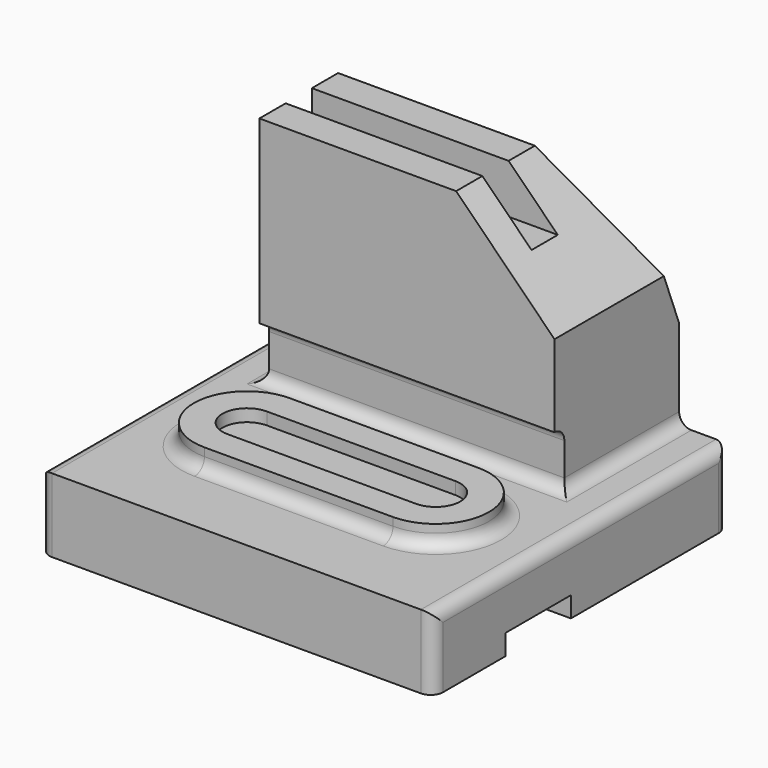
from build123d import *

# Parameters (mm, degrees)
F0_W      = 96
F0_H      = 90
F1_DEPTH  = 18
F2_W      = 72
F2_H      = 38
F4_DEPTH  = 58
F6_DEPTH  = 38
F7_W      = 8
F7_H      = 12
F8_DEPTH  = 60.001
F10_DEPTH = 72.001
F11_W     = 20
F11_H     = 5
F12_DEPTH = 96
F13_W     = 46
F13_H     = 26
F14_DEPTH = 5
F15_W     = 46
F15_H     = 12
F17_DEPTH = 3
F18_W     = 3
F18_H     = 14
F19_DEPTH = 72
F20_R     = 2.99999


# Not quite as in the source:
# - a fillet or chamfer is up to 0.001 mm smaller than in the source, because OpenCascade refuses the exact size


with BuildPart() as f1:
    # F0 (on Top) → F1 (new body)
    with BuildSketch(Plane.XY):
        with Locations((48, 45)):
            Rectangle(F0_W, F0_H)
    extrude(amount=F1_DEPTH)

    # F2 (on face) → F4 (join, through all)
    with BuildSketch(Plane.XY.offset(18)):
        with Locations((48, 71)):
            Rectangle(F2_W, F2_H)
    extrude(amount=F4_DEPTH)

    # F5 (on face) → F6 (cut, through all)
    with BuildSketch(Plane.XZ.offset(-52)):
        Polygon((84, 52), (84, 76), (60, 76), align=None)
    extrude(amount=-F6_DEPTH, mode=Mode.SUBTRACT)

    # F7 (on face) → F8 (cut, through all)
    with BuildSketch(Plane(origin=(12, 0, 0), x_dir=(0, -1, 0), z_dir=(-1, 0, 0))):
        with Locations((-64, 70)):
            Rectangle(F7_W, F7_H)
    extrude(amount=-F8_DEPTH, mode=Mode.SUBTRACT)

    # F9 (on face) → F10 (cut, through all)
    with BuildSketch(Plane(origin=(12, 0, 0), x_dir=(0, -1, 0), z_dir=(-1, 0, 0))):
        Polygon((-90, 40), (-76, 76), (-90, 76), align=None)
    extrude(amount=-F10_DEPTH, mode=Mode.SUBTRACT)

    # F11 (on face) → F12 (cut, through all)
    with BuildSketch(Plane.YZ.offset(96)):
        with Locations((32, 2.5)):
            Rectangle(F11_W, F11_H)
    extrude(amount=-F12_DEPTH, mode=Mode.SUBTRACT)

    # F13 (on face) → F14 (join)
    with BuildSketch(Plane.XY.offset(18)):
        with Locations((48, 31.9999999999)):
            Rectangle(F13_W, F13_H)
        with BuildLine():
            Line((25, 18.9999999999), (25, 44.9999999999))
            ThreePointArc((25, 44.9999999999), (12, 31.9999999999), (25, 18.9999999999))
        make_face()
        with BuildLine():
            ThreePointArc((71, 18.9999999999), (84, 31.9999999999), (71, 44.9999999999))
            Line((71, 44.9999999999), (71, 18.9999999999))
        make_face()
    extrude(amount=F14_DEPTH)

    # F15 (on face) → F17 (cut, through all)
    with BuildSketch(Plane.XY.offset(23)):
        with Locations((48, 31.9999999999)):
            Rectangle(F15_W, F15_H)
        with BuildLine():
            Line((25, 25.9999999999), (25, 37.9999999999))
            ThreePointArc((25, 37.9999999999), (19, 31.9999999999), (25, 25.9999999999))
        make_face()
        with BuildLine():
            ThreePointArc((71, 25.9999999999), (77, 31.9999999999), (71, 37.9999999999))
            Line((71, 37.9999999999), (71, 25.9999999999))
        make_face()
    extrude(amount=-F17_DEPTH, mode=Mode.SUBTRACT)

    # F18 (on face) → F19 (cut, through all)
    with BuildSketch(Plane.YZ.offset(84)):
        with Locations((53.5, 25)):
            Rectangle(F18_W, F18_H)
    extrude(amount=-F19_DEPTH, mode=Mode.SUBTRACT)

    # F20 (radius 3 in the source; OpenCascade refuses exactly that, so slightly less here)
    f20_edges = [f1.edges().sort_by_distance(p)[0] for p in [
        (48, 19, 18),
        (48, 55, 18),
        (48, 55, 32),
        (84, 72.5, 18),
        (12, 72.5, 18),
        (0, 45, 18),
        (96, 45, 18),
        (96, 0, 9),
        (0, 0, 9),
        (0, 90, 9),
        (96, 90, 9),
    ]]
    fillet(f20_edges, radius=F20_R)


solid = f1.part
